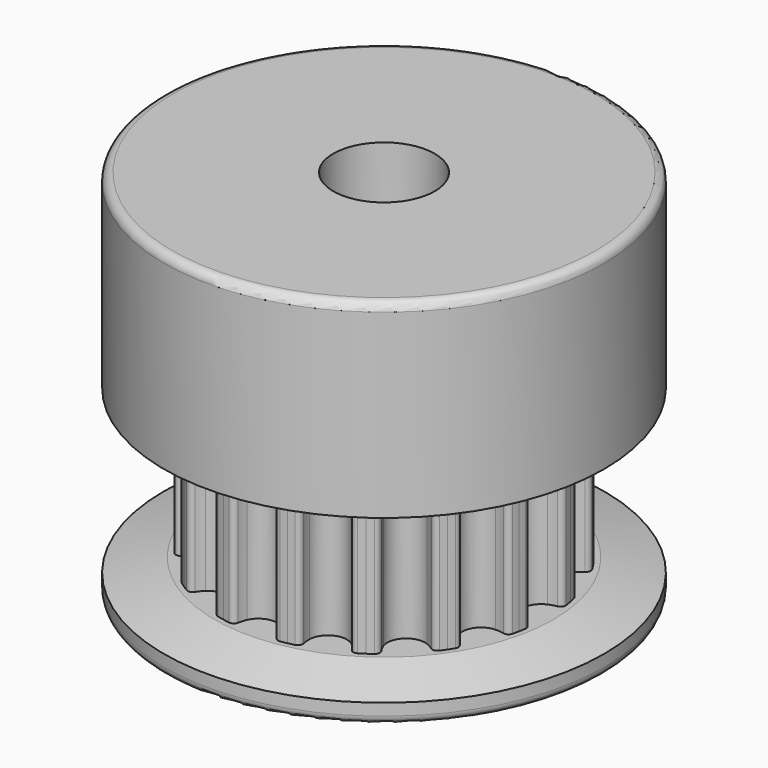
from build123d import *

# Parameters (mm, degrees)
F3_DEPTH    = 2
F4_COUNT    = 16
F5_R        = 6.5
F6_DEPTH    = 1
F7_R        = 6.5
F8_DEPTH    = 1
F9_R        = 6.5
F10_DEPTH   = 5
F11_R       = 1.5
F12_DEPTH   = 11.001
F13_R       = 1.5
F14_DEPTH   = 6.501
F15_R       = 1.5
F16_DEPTH   = 6.5010001
F17_SIZE2   = 0.4019237886
F17_SIZE    = 1.5
F17_2_SIZE2 = 0.4019237886
F17_2_SIZE  = 1.5
F18_R       = 0.25


# Not quite as in the source:
# - a feature names something its author has since deleted; it is built from what else it names


with BuildPart() as f3:
    # F2 (on Top) → F3 (new body, symmetric)
    with BuildSketch(Plane.XY):
        with BuildLine():
            ThreePointArc((0.5070084573, 4.4150779199), (0.3022651059, 4.1753692078), (0, 4.0858375803))
            ThreePointArc((0, 4.0858375803), (-0.3022651059, 4.1753692078), (-0.5070084573, 4.4150779199))
            ThreePointArc((-0.5070084573, 4.4150779199), (-0.5510572691, 4.5336764254), (-0.5797791871, 4.6568874426))
            ThreePointArc((-0.5797791871, 4.6568874426), (-0.6400054613, 4.7538203484), (-0.7510040389, 4.7803252181))
            ThreePointArc((-0.7510040389, 4.7803252181), (-0.8476929444, 4.7641298187), (-0.9440339094, 4.7459789544))
            Line((-0.9440339094, 4.7459789544), (0, 0))
            Line((0, 0), (0.9440339094, 4.7459789544))
            ThreePointArc((0.9440339094, 4.7459789544), (0.8476929444, 4.7641298187), (0.7510040389, 4.7803252181))
            ThreePointArc((0.7510040389, 4.7803252181), (0.6400054613, 4.7538203484), (0.5797791871, 4.6568874426))
            ThreePointArc((0.5797791871, 4.6568874426), (0.5510572691, 4.5336764254), (0.5070084573, 4.4150779199))
        make_face()
    extrude(amount=F3_DEPTH, both=True)

    # F4: F3 ×16 about axis
    f4_axis = Axis((0, 0, 0), (0, 0, -1))


with BuildPart() as f3_1:
    add(f3.part)
    for i in range(1, F4_COUNT):
        add(f3.part.rotate(f4_axis, i * 360 / F4_COUNT))

    # F5 (on face) → F6 (join)
    with BuildSketch(Plane(origin=(0, 0, -2), x_dir=(1, 0, 0), z_dir=(0, 0, -1))):
        Circle(F5_R)
    extrude(amount=F6_DEPTH)

    # F7 (on face) → F8 (join)
    with BuildSketch(Plane.XY.offset(2)):
        Circle(F7_R)
    extrude(amount=F8_DEPTH)

    # F9 (on face) → F10 (join)
    with BuildSketch(Plane.XY.offset(3)):
        Circle(F9_R)
    extrude(amount=F10_DEPTH)

    # F11 (on face) → F12 (cut, through all)
    with BuildSketch(Plane.XY.offset(8)):
        Circle(F11_R)
    extrude(amount=-F12_DEPTH, mode=Mode.SUBTRACT)

    # F13 (on Front) → F14 (cut, through all)
    with BuildSketch(Plane.XZ):
        with Locations((0, 5)):
            Circle(F13_R)
    extrude(amount=-F14_DEPTH, mode=Mode.SUBTRACT)

    # F15 (on Right) → F16 (cut, through all)
    with BuildSketch(Plane.YZ):
        with Locations((0, 5)):
            Circle(F15_R)
    extrude(amount=-F16_DEPTH, mode=Mode.SUBTRACT)

    # F17
    f17_edges = [f3_1.edges().sort_by_distance(p)[0] for p in [
        (-6.5, 0, -2),
    ]]
    f17_side = f3_1.faces().sort_by_distance((-6.316152, 0, -2))[0]
    chamfer(f17_edges, length=F17_SIZE, length2=F17_SIZE2, reference=f17_side)

    # F17#2
    f17_2_edges = [f3_1.edges().sort_by_distance(p)[0] for p in [
        (-6.5, 0, 2),
    ]]
    f17_2_side = f3_1.faces().sort_by_distance((-6.316152, 0, 2))[0]
    chamfer(f17_2_edges, length=F17_2_SIZE, length2=F17_2_SIZE2, reference=f17_2_side)

    # F18
    f18_edges = [f3_1.edges().sort_by_distance(p)[0] for p in [
        (-6.5, 0, 8),
        (-6.5, 0, -3),
    ]]
    fillet(f18_edges, radius=F18_R)


solid = f3_1.part
